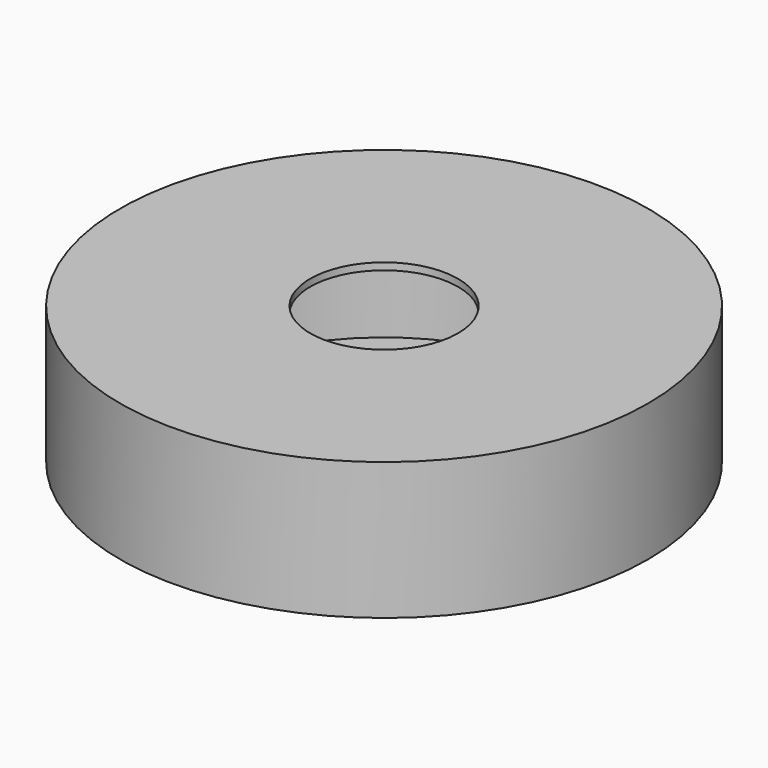
from build123d import *

# Parameters (mm, degrees)
F0_R     = 15
F0_R_2   = 11.2
F1_DEPTH = 3.5
F2_R     = 15
F3_DEPTH = 0.4
F4_R     = 4.2
F5_DEPTH = 7.801


# Not quite as in the source:
# - a pattern or mirror of a feature is missing from the dataset's text; its kind, count and spacing are read off the source's solid


with BuildPart() as f1:
    # F0 (on Top) → F1 (new body, symmetric)
    with BuildSketch(Plane.XY):
        Circle(F0_R)
        Circle(F0_R_2, mode=Mode.SUBTRACT)
    extrude(amount=F1_DEPTH, both=True)

    # F2 (on face) → F3 (join)
    with BuildSketch(Plane(origin=(0, 0, -3.5), x_dir=(1, 0, 0), z_dir=(0, 0, -1))):
        Circle(F2_R)
    f3 = extrude(amount=F3_DEPTH)

    # F3_copies: F3 across plane
    add(f3.mirror(Plane.XY))

    # F4 (on face) → F5 (cut, through all)
    with BuildSketch(Plane(origin=(0, 0, -3.9), x_dir=(1, 0, 0), z_dir=(0, 0, -1))):
        Circle(F4_R)
    extrude(amount=-F5_DEPTH, mode=Mode.SUBTRACT)


solid = f1.part
